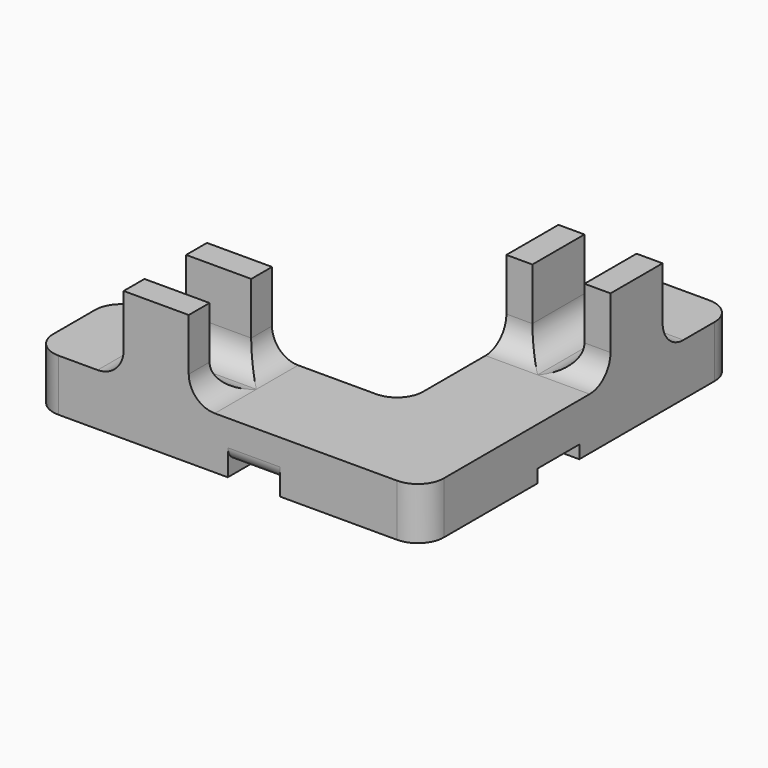
from build123d import *

# Parameters (mm, degrees)
F1_DEPTH = 4
F2_W     = 2
F2_H     = 5
F2_W_2   = 5
F2_H_2   = 2
F3_DEPTH = 6
F4_R     = 1.99999
F5_W     = 4
F5_H     = 1
F6_DEPTH = 25
F7_R     = 1
F8_W     = 4
F8_H     = 1
F9_DEPTH = 25


# Not quite as in the source:
# - a fillet or chamfer is up to 0.001 mm smaller than in the source, because OpenCascade refuses the exact size


with BuildPart() as f1:
    # F0 (on Top) → F1 (new body)
    with BuildSketch(Plane.XY):
        Polygon((8, -8), (8, 22), (0, 22), (0, 0), (-22, 0), (-22, -8), align=None)
    extrude(amount=F1_DEPTH)

    # F2 (on face) → F3 (join)
    with BuildSketch(Plane.XY.offset(4)):
        with Locations((1, 12.5)):
            Rectangle(F2_W, F2_H)
        with Locations((7, 12.5)):
            Rectangle(F2_W, F2_H)
        with Locations((-12.5, -1)):
            Rectangle(F2_W_2, F2_H_2)
        with Locations((-12.5, -7)):
            Rectangle(F2_W_2, F2_H_2)
    extrude(amount=F3_DEPTH)

    # F4 (radius 2 in the source; OpenCascade refuses exactly that, so slightly less here)
    f4_edges = [f1.edges().sort_by_distance(p)[0] for p in [
        (1, 15, 4),
        (2, 12.5, 4),
        (7, 15, 4),
        (-12.5, -6, 4),
        (-10, -7, 4),
        (1, 10, 4),
        (7, 10, 4),
        (6, 12.5, 4),
        (-15, -7, 4),
        (0, 0, 2),
        (8, -8, 2),
        (-15, -1, 4),
        (-12.5, -2, 4),
        (-10, -1, 4),
        (8, 22, 2),
        (0, 22, 2),
        (-22, -8, 2),
        (-22, 0, 2),
    ]]
    fillet(f4_edges, radius=F4_R)

    # F5 (on face) → F6 (cut)
    with BuildSketch(Plane.XZ.offset(8)):
        with Locations((-5, 0.5)):
            Rectangle(F5_W, F5_H)
    extrude(amount=-F6_DEPTH, mode=Mode.SUBTRACT)

    # F7
    f7_edges = [f1.edges().sort_by_distance(p)[0] for p in [
        (-5, -8, 1),
        (-5, 0, 1),
    ]]
    fillet(f7_edges, radius=F7_R)

    # F8 (on face) → F9 (cut)
    with BuildSketch(Plane.YZ.offset(8)):
        with Locations((5, 0.5)):
            Rectangle(F8_W, F8_H)
    extrude(amount=-F9_DEPTH, mode=Mode.SUBTRACT)


solid = f1.part
